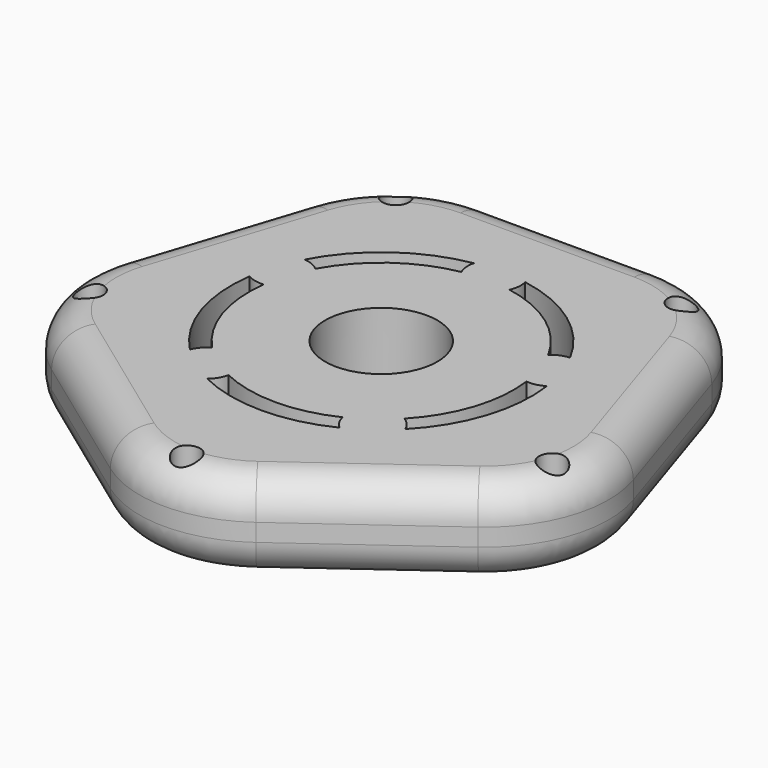
from build123d import *

# Parameters (mm, degrees)
F0_R         = 0.75
F0_R_2       = 3.175
F1_DEPTH     = 5
F2_R         = 7
F3_T1_DEPTH  = 9.8284046079
F3_T3_DEPTH  = 9.8284046079
F3_T5_DEPTH  = 9.8284046079
F3_T7_DEPTH  = 9.8284046079
F3_T9_DEPTH  = 9.8284046079
F3_T12_ANGLE = 72
F3_T14_ANGLE = 72
F3_T16_ANGLE = 72
F3_T18_ANGLE = 72
F3_T20_ANGLE = 72
F4_T1_DEPTH  = 9.8284046079
F4_T3_DEPTH  = 9.8284046079
F4_T5_DEPTH  = 9.8284046079
F4_T7_DEPTH  = 9.8284046079
F4_T9_DEPTH  = 9.8284046079
F4_T12_ANGLE = 72
F4_T14_ANGLE = 72
F4_T16_ANGLE = 72
F4_T18_ANGLE = 72
F4_T20_ANGLE = 72


# Not quite as in the source:
# - a fillet or chamfer that OpenCascade refuses, or shapes differently, is made with other operations: its cross-section is extruded or revolved along the edge and cut away or added


with BuildPart() as f1:
    # F0 (on Top) → F1 (new body)
    with BuildSketch(Plane.XY):
        Polygon((10, 13.7638192047), (-10, 13.7638192047), (-16.1803398875, -5.2573111212), (0, -17.013016167), (16.1803398875, -5.2573111212), align=None)
        with Locations((-13.0901699437, -4.2532540418)):
            Circle(F0_R, mode=Mode.SUBTRACT)
        with BuildLine():
            ThreePointArc((-6.0976924927, -5.9218363929), (-8.0839803885, -2.6266444522), (-8.4139049513, 1.2067325595))
            ThreePointArc((-8.4139049513, 1.2067325595), (-7.944006, 1.0101497716), (-7.4354139864, 0.9821501159))
            ThreePointArc((-7.4354139864, 0.9821501159), (-7.1329238722, -2.3176274578), (-5.4380829216, -5.1650028207))
            ThreePointArc((-5.4380829216, -5.1650028207), (-5.8330847191, -5.486597903), (-6.0976924927, -5.9218363929))
        make_face(mode=Mode.SUBTRACT)
        with Locations((0, -13.7638192047)):
            Circle(F0_R, mode=Mode.SUBTRACT)
        with BuildLine():
            ThreePointArc((-3.2317495497, -6.7679978463), (0, -7.5), (3.2317495497, -6.7679978463))
            ThreePointArc((3.2317495497, -6.7679978463), (3.4155423801, -7.2430452255), (3.7477104832, -7.6291982629))
            ThreePointArc((3.7477104832, -7.6291982629), (0, -8.5), (-3.7477104832, -7.6291982629))
            ThreePointArc((-3.7477104832, -7.6291982629), (-3.4155423801, -7.2430452255), (-3.2317495497, -6.7679978463))
        make_face(mode=Mode.SUBTRACT)
        with BuildLine():
            ThreePointArc((5.4380829216, -5.1650028207), (7.1329238722, -2.3176274578), (7.4354139864, 0.9821501159))
            ThreePointArc((7.4354139864, 0.9821501159), (7.944006, 1.0101497716), (8.4139049513, 1.2067325595))
            ThreePointArc((8.4139049513, 1.2067325595), (8.0839803885, -2.6266444522), (6.0976924927, -5.9218363929))
            ThreePointArc((6.0976924927, -5.9218363929), (5.8330847191, -5.486597903), (5.4380829216, -5.1650028207))
        make_face(mode=Mode.SUBTRACT)
        with Locations((13.0901699437, -4.2532540418)):
            Circle(F0_R, mode=Mode.SUBTRACT)
        with BuildLine():
            ThreePointArc((-1.4523687548, 8.375), (-1.4941233347, 7.8673521181), (-1.3635890143, 7.375))
            ThreePointArc((-1.3635890143, 7.375), (-4.4083893922, 6.0676274578), (-6.5926696289, 3.5758505511))
            ThreePointArc((-6.5926696289, 3.5758505511), (-7.0205869958, 3.8521412389), (-7.5162916966, 3.9693020962))
            ThreePointArc((-7.5162916966, 3.9693020962), (-4.9961746445, 6.8766444522), (-1.4523687548, 8.375))
        make_face(mode=Mode.SUBTRACT)
        with Locations((-8.0901699437, 11.1351636441)):
            Circle(F0_R, mode=Mode.SUBTRACT)
        Circle(F0_R_2, mode=Mode.SUBTRACT)
        with BuildLine():
            ThreePointArc((6.5926696289, 3.5758505511), (4.4083893922, 6.0676274578), (1.3635890143, 7.375))
            ThreePointArc((1.3635890143, 7.375), (1.4941233347, 7.8673521181), (1.4523687548, 8.375))
            ThreePointArc((1.4523687548, 8.375), (4.9961746445, 6.8766444522), (7.5162916966, 3.9693020962))
            ThreePointArc((7.5162916966, 3.9693020962), (7.0205869958, 3.8521412389), (6.5926696289, 3.5758505511))
        make_face(mode=Mode.SUBTRACT)
        with Locations((8.0901699437, 11.1351636441)):
            Circle(F0_R, mode=Mode.SUBTRACT)
    extrude(amount=F1_DEPTH)

    # F2
    f2_edges = [f1.edges().sort_by_distance(p)[0] for p in [
        (16.18034, -5.257311, 2.5),
        (10, 13.763819, 2.5),
        (-10, 13.763819, 2.5),
        (-16.18034, -5.257311, 2.5),
        (0, -17.013016, 2.5),
    ]]
    fillet(f2_edges, radius=F2_R)

    # F3: fillet of radius 2 on 10 edges, made by hand

    # F3_s2 → F3_t1 (cut)
    with BuildSketch(Plane.YZ.offset(-4.914202304)):
        with BuildLine():
            ThreePointArc((13.7638192047, 2), (13.1780327671, 0.5857864376), (11.7638192047, 0))
            Line((11.7638192047, 0), (13.7638192047, 0))
            Line((13.7638192047, 0), (13.7638192047, 2))
        make_face()
    extrude(amount=F3_T1_DEPTH, mode=Mode.SUBTRACT)

    # F3_s4 → F3_t3 (cut)
    with BuildSketch(Plane(origin=(1.5185720257, -4.6736841236, 0), x_dir=(0, 0, 1), z_dir=(-0.3090169944, 0.9510565163, 0))):
        with BuildLine():
            ThreePointArc((0, 11.7638192047), (0.5857864376, 13.1780327671), (2, 13.7638192047))
            Line((2, 13.7638192047), (0, 13.7638192047))
            Line((0, 13.7638192047), (0, 11.7638192047))
        make_face()
    extrude(amount=F3_T3_DEPTH, mode=Mode.SUBTRACT)

    # F3_s6 → F3_t5 (cut)
    with BuildSketch(Plane(origin=(-3.9756731777, -2.8884956411, 0), x_dir=(0, 0, 1), z_dir=(0.8090169944, 0.5877852523, 0))):
        with BuildLine():
            ThreePointArc((0, 11.7638192047), (0.5857864376, 13.1780327671), (2, 13.7638192047))
            Line((2, 13.7638192047), (0, 13.7638192047))
            Line((0, 13.7638192047), (0, 11.7638192047))
        make_face()
    extrude(amount=F3_T5_DEPTH, mode=Mode.SUBTRACT)

    # F3_s8 → F3_t7 (cut)
    with BuildSketch(Plane(origin=(-3.9756731777, 2.8884956411, 0), x_dir=(0, 0, 1), z_dir=(0.8090169944, -0.5877852523, 0))):
        with BuildLine():
            ThreePointArc((0, 11.7638192047), (0.5857864376, 13.1780327671), (2, 13.7638192047))
            Line((2, 13.7638192047), (0, 13.7638192047))
            Line((0, 13.7638192047), (0, 11.7638192047))
        make_face()
    extrude(amount=F3_T7_DEPTH, mode=Mode.SUBTRACT)

    # F3_s10 → F3_t9 (cut)
    with BuildSketch(Plane(origin=(1.5185720257, 4.6736841236, 0), x_dir=(0, 0, 1), z_dir=(-0.3090169944, -0.9510565163, 0))):
        with BuildLine():
            ThreePointArc((0, 11.7638192047), (0.5857864376, 13.1780327671), (2, 13.7638192047))
            Line((2, 13.7638192047), (0, 13.7638192047))
            Line((0, 13.7638192047), (0, 11.7638192047))
        make_face()
    extrude(amount=F3_T9_DEPTH, mode=Mode.SUBTRACT)

    # F3_s11 → F3_t12 (revolve, cut)
    with BuildSketch(Plane.YZ.offset(4.914202304)):
        with BuildLine():
            ThreePointArc((11.7638192047, 0), (13.1780327671, 0.5857864376), (13.7638192047, 2))
            Line((13.7638192047, 2), (13.7638192047, 0))
            Line((13.7638192047, 0), (11.7638192047, 0))
        make_face()
    revolve(axis=Axis((4.914202304, 6.7638192047, 0), (0, 0, -1)), revolution_arc=F3_T12_ANGLE, mode=Mode.SUBTRACT)

    # F3_s13 → F3_t14 (revolve, cut)
    with BuildSketch(Plane(origin=(3.9756731777, 2.8884956411, 0), x_dir=(0, 0, 1), z_dir=(-0.8090169944, -0.5877852523, 0))):
        with BuildLine():
            ThreePointArc((0, -11.7638192047), (0.5857864376, -13.1780327671), (2, -13.7638192047))
            Line((2, -13.7638192047), (0, -13.7638192047))
            Line((0, -13.7638192047), (0, -11.7638192047))
        make_face()
    revolve(axis=Axis((7.9513463554, -2.5835490424, 0), (0, 0, 1)), revolution_arc=F3_T14_ANGLE, mode=Mode.SUBTRACT)

    # F3_s15 → F3_t16 (revolve, cut)
    with BuildSketch(Plane(origin=(3.9756731777, -2.8884956411, 0), x_dir=(0, 0, 1), z_dir=(-0.8090169944, 0.5877852523, 0))):
        with BuildLine():
            ThreePointArc((0, -11.7638192047), (0.5857864376, -13.1780327671), (2, -13.7638192047))
            Line((2, -13.7638192047), (0, -13.7638192047))
            Line((0, -13.7638192047), (0, -11.7638192047))
        make_face()
    revolve(axis=Axis((0, -8.3605403245, 0), (0, 0, 1)), revolution_arc=F3_T16_ANGLE, mode=Mode.SUBTRACT)

    # F3_s17 → F3_t18 (revolve, cut)
    with BuildSketch(Plane(origin=(-1.5185720257, -4.6736841236, 0), x_dir=(0, 0, 1), z_dir=(0.3090169944, 0.9510565163, 0))):
        with BuildLine():
            ThreePointArc((0, -11.7638192047), (0.5857864376, -13.1780327671), (2, -13.7638192047))
            Line((2, -13.7638192047), (0, -13.7638192047))
            Line((0, -13.7638192047), (0, -11.7638192047))
        make_face()
    revolve(axis=Axis((-7.9513463554, -2.5835490424, 0), (0, 0, 1)), revolution_arc=F3_T18_ANGLE, mode=Mode.SUBTRACT)

    # F3_s19 → F3_t20 (revolve, cut)
    with BuildSketch(Plane.YZ.offset(-4.914202304)):
        with BuildLine():
            ThreePointArc((11.7638192047, 0), (13.1780327671, 0.5857864376), (13.7638192047, 2))
            Line((13.7638192047, 2), (13.7638192047, 0))
            Line((13.7638192047, 0), (11.7638192047, 0))
        make_face()
    revolve(axis=Axis((-4.914202304, 6.7638192047, 0), (0, 0, 1)), revolution_arc=F3_T20_ANGLE, mode=Mode.SUBTRACT)

    # F4: fillet of radius 2 on 10 edges, made by hand

    # F4_s2 → F4_t1 (cut)
    with BuildSketch(Plane.YZ.offset(-4.914202304)):
        with BuildLine():
            ThreePointArc((13.7638192047, 3), (13.1780327671, 4.4142135624), (11.7638192047, 5))
            Line((11.7638192047, 5), (13.7638192047, 5))
            Line((13.7638192047, 5), (13.7638192047, 3))
        make_face()
    extrude(amount=F4_T1_DEPTH, mode=Mode.SUBTRACT)

    # F4_s4 → F4_t3 (cut)
    with BuildSketch(Plane(origin=(1.5185720257, -4.6736841236, 0), x_dir=(0, 0, 1), z_dir=(-0.3090169944, 0.9510565163, 0))):
        with BuildLine():
            ThreePointArc((5, 11.7638192047), (4.4142135624, 13.1780327671), (3, 13.7638192047))
            Line((3, 13.7638192047), (5, 13.7638192047))
            Line((5, 13.7638192047), (5, 11.7638192047))
        make_face()
    extrude(amount=F4_T3_DEPTH, mode=Mode.SUBTRACT)

    # F4_s6 → F4_t5 (cut)
    with BuildSketch(Plane(origin=(-3.9756731777, -2.8884956411, 0), x_dir=(0, 0, 1), z_dir=(0.8090169944, 0.5877852523, 0))):
        with BuildLine():
            ThreePointArc((5, 11.7638192047), (4.4142135624, 13.1780327671), (3, 13.7638192047))
            Line((3, 13.7638192047), (5, 13.7638192047))
            Line((5, 13.7638192047), (5, 11.7638192047))
        make_face()
    extrude(amount=F4_T5_DEPTH, mode=Mode.SUBTRACT)

    # F4_s8 → F4_t7 (cut)
    with BuildSketch(Plane(origin=(1.5185720257, 4.6736841236, 0), x_dir=(0, 0, 1), z_dir=(-0.3090169944, -0.9510565163, 0))):
        with BuildLine():
            ThreePointArc((5, 11.7638192047), (4.4142135624, 13.1780327671), (3, 13.7638192047))
            Line((3, 13.7638192047), (5, 13.7638192047))
            Line((5, 13.7638192047), (5, 11.7638192047))
        make_face()
    extrude(amount=F4_T7_DEPTH, mode=Mode.SUBTRACT)

    # F4_s10 → F4_t9 (cut)
    with BuildSketch(Plane(origin=(-3.9756731777, 2.8884956411, 0), x_dir=(0, 0, 1), z_dir=(0.8090169944, -0.5877852523, 0))):
        with BuildLine():
            ThreePointArc((5, 11.7638192047), (4.4142135624, 13.1780327671), (3, 13.7638192047))
            Line((3, 13.7638192047), (5, 13.7638192047))
            Line((5, 13.7638192047), (5, 11.7638192047))
        make_face()
    extrude(amount=F4_T9_DEPTH, mode=Mode.SUBTRACT)

    # F4_s11 → F4_t12 (revolve, cut)
    with BuildSketch(Plane.YZ.offset(4.914202304)):
        with BuildLine():
            ThreePointArc((11.7638192047, 5), (13.1780327671, 4.4142135624), (13.7638192047, 3))
            Line((13.7638192047, 3), (13.7638192047, 5))
            Line((13.7638192047, 5), (11.7638192047, 5))
        make_face()
    revolve(axis=Axis((4.914202304, 6.7638192047, 5), (0, 0, -1)), revolution_arc=F4_T12_ANGLE, mode=Mode.SUBTRACT)

    # F4_s13 → F4_t14 (revolve, cut)
    with BuildSketch(Plane.YZ.offset(-4.914202304)):
        with BuildLine():
            ThreePointArc((13.7638192047, 3), (13.1780327671, 4.4142135624), (11.7638192047, 5))
            Line((11.7638192047, 5), (13.7638192047, 5))
            Line((13.7638192047, 5), (13.7638192047, 3))
        make_face()
    revolve(axis=Axis((-4.914202304, 6.7638192047, 5), (0, 0, 1)), revolution_arc=F4_T14_ANGLE, mode=Mode.SUBTRACT)

    # F4_s15 → F4_t16 (revolve, cut)
    with BuildSketch(Plane(origin=(3.9756731777, 2.8884956411, 0), x_dir=(0, 0, 1), z_dir=(-0.8090169944, -0.5877852523, 0))):
        with BuildLine():
            ThreePointArc((5, -11.7638192047), (4.4142135624, -13.1780327671), (3, -13.7638192047))
            Line((3, -13.7638192047), (5, -13.7638192047))
            Line((5, -13.7638192047), (5, -11.7638192047))
        make_face()
    revolve(axis=Axis((7.9513463554, -2.5835490424, 5), (0, 0, 1)), revolution_arc=F4_T16_ANGLE, mode=Mode.SUBTRACT)

    # F4_s17 → F4_t18 (revolve, cut)
    with BuildSketch(Plane(origin=(3.9756731777, -2.8884956411, 0), x_dir=(0, 0, 1), z_dir=(-0.8090169944, 0.5877852523, 0))):
        with BuildLine():
            ThreePointArc((5, -11.7638192047), (4.4142135624, -13.1780327671), (3, -13.7638192047))
            Line((3, -13.7638192047), (5, -13.7638192047))
            Line((5, -13.7638192047), (5, -11.7638192047))
        make_face()
    revolve(axis=Axis((0, -8.3605403245, 5), (0, 0, 1)), revolution_arc=F4_T18_ANGLE, mode=Mode.SUBTRACT)

    # F4_s19 → F4_t20 (revolve, cut)
    with BuildSketch(Plane(origin=(-1.5185720257, -4.6736841236, 0), x_dir=(0, 0, 1), z_dir=(0.3090169944, 0.9510565163, 0))):
        with BuildLine():
            ThreePointArc((5, -11.7638192047), (4.4142135624, -13.1780327671), (3, -13.7638192047))
            Line((3, -13.7638192047), (5, -13.7638192047))
            Line((5, -13.7638192047), (5, -11.7638192047))
        make_face()
    revolve(axis=Axis((-7.9513463554, -2.5835490424, 5), (0, 0, 1)), revolution_arc=F4_T20_ANGLE, mode=Mode.SUBTRACT)


solid = f1.part
